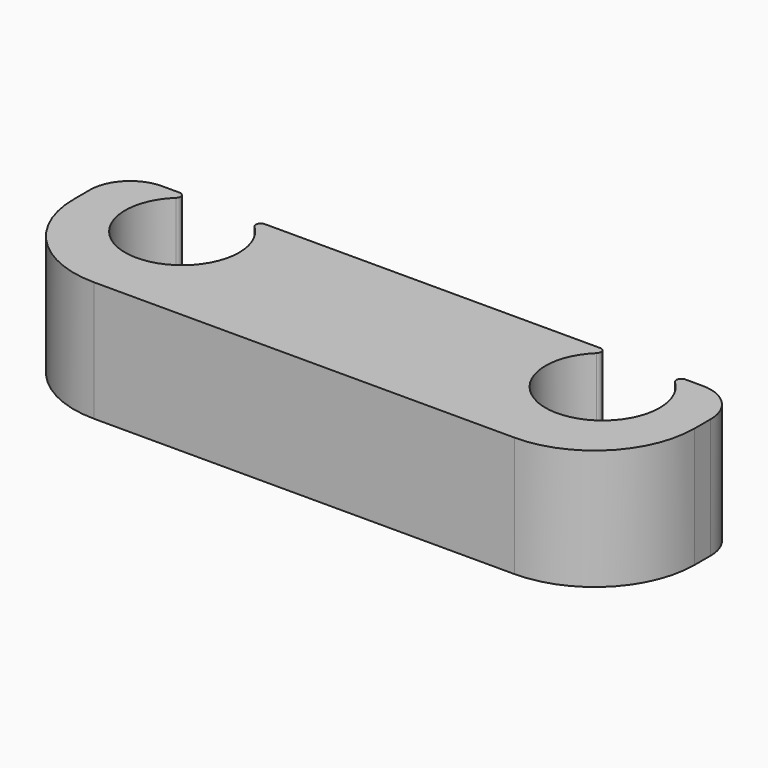
from build123d import *

# Parameters (mm, degrees)
F1_DEPTH = 6
F2_R     = 5
F3_R     = 2
F4_R     = 0.25


with BuildPart() as f1:
    # F0 (on Top) → F1 (new body)
    with BuildSketch(Plane.XY):
        with BuildLine():
            Line((-11.8683932183, 4), (-15.5, 4))
            Line((-15.5, 4), (-15.5, -4))
            Line((-15.5, -4), (15.5, -4))
            Line((15.5, -4), (15.5, 4))
            Line((15.5, 4), (11.8683932183, 4))
            ThreePointArc((11.8683932183, 4), (12.9517769752, 2.9530277574), (13.35, 1.5))
            ThreePointArc((13.35, 1.5), (9.0469722426, -0.9517769752), (9.1316067817, 4))
            Line((9.1316067817, 4), (-9.1316067817, 4))
            ThreePointArc((-9.1316067817, 4), (-8.0482230248, 2.9530277574), (-7.65, 1.5))
            ThreePointArc((-7.65, 1.5), (-11.9530277574, -0.9517769752), (-11.8683932183, 4))
        make_face()
    extrude(amount=F1_DEPTH)

    # F2
    f2_edges = [f1.edges().sort_by_distance(p)[0] for p in [
        (15.5, -4, 3),
        (-15.5, -4, 3),
    ]]
    fillet(f2_edges, radius=F2_R)

    # F3
    f3_edges = [f1.edges().sort_by_distance(p)[0] for p in [
        (-15.5, 4, 3),
        (15.5, 4, 3),
    ]]
    fillet(f3_edges, radius=F3_R)

    # F4
    f4_edges = [f1.edges().sort_by_distance(p)[0] for p in [
        (9.131607, 4, 3),
        (11.868393, 4, 3),
        (-9.131607, 4, 3),
        (-11.868393, 4, 3),
    ]]
    fillet(f4_edges, radius=F4_R)


solid = f1.part
